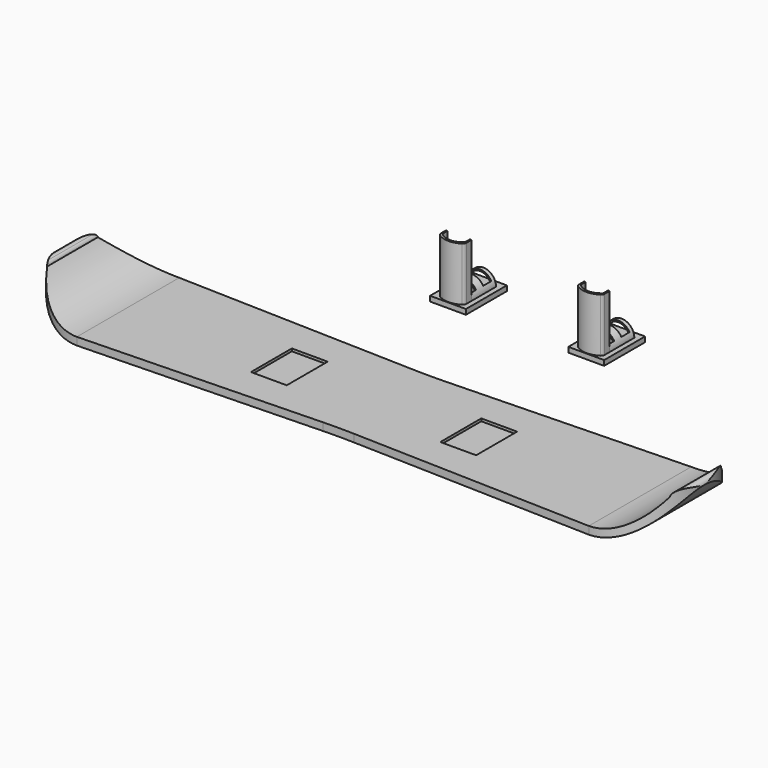
from build123d import *

# Parameters (mm, degrees)
F1_DEPTH    = 9.8425
F3_DEPTH    = 25.4
F5_DEPTH    = 2.667
F6_T1_DEPTH = 0.381
F0_W        = 1.778
F0_H        = 2.54
F0_W_2      = 1.1176
F0_H_2      = 0.508
F0_H_3      = 0.4445
F0_H_4      = 0.2032
F0_W_3      = 0.0762
F0_H_5      = 0.6812858045
F7_DEPTH    = 2.921
F8_DEPTH    = 2.667
F9_DEPTH    = 2.667
F12_DEPTH   = 1.524


# Not quite as in the source:
# - a fillet or chamfer that OpenCascade refuses, or shapes differently, is made with other operations: its cross-section is extruded or revolved along the edge and cut away or added


with BuildPart() as f1:
    # F0 (on Top) → F1 (new body)
    with BuildSketch(Plane.XY):
        with BuildLine():
            Line((-12.7, -6.35), (-12.7, 0))
            ThreePointArc((-12.7, 0), (-15.875, -3.175), (-12.7, -6.35))
        make_face()
        with BuildLine():
            ThreePointArc((12.7, -6.35), (15.875, -3.175), (12.7, 0))
            Line((12.7, 0), (12.7, -6.35))
        make_face()
        Polygon((-6.35, -0.1905), (-12.7, 0), (-12.7, -6.35), (-6.35, -6.1595), (0, -5.969), (6.35, -6.1595), (12.7, -6.35), (12.7, 0), (6.35, -0.1905), (0, -0.381), align=None)
    extrude(amount=-F1_DEPTH)

    # F2 (on Front) → F3 (cut)
    with BuildSketch(Plane.XZ):
        with BuildLine():
            Line((-12.7, -2.54), (0, -2.54))
            Line((0, -2.54), (12.7, -2.54))
            ThreePointArc((12.7, -2.54), (14.2747487895, -2.1336283165), (15.4562218706, -1.016))
            ThreePointArc((15.4562218706, -1.016), (15.4848358871, -0.9182319253), (15.5561717457, -0.8455094828))
            ThreePointArc((15.5561717457, -0.8455094828), (15.745074667, -0.4338744994), (15.875, 0))
            Line((15.875, 0), (-15.875, 0))
            ThreePointArc((-15.875, 0), (-15.7450242413, -0.4340082159), (-15.556034737, -0.8457603215))
            ThreePointArc((-15.556034737, -0.8457603215), (-15.484834563, -0.9183954726), (-15.4562218706, -1.016))
            ThreePointArc((-15.4562218706, -1.016), (-14.2747487895, -2.1336283165), (-12.7, -2.54))
        make_face()
        with BuildLine():
            ThreePointArc((-15.875, -1.016), (-15.7642823045, -0.8395129732), (-15.556034737, -0.8457603215))
            ThreePointArc((-15.556034737, -0.8457603215), (-15.7450242413, -0.4340082159), (-15.875, 0))
            Line((-15.875, 0), (-15.875, -1.016))
        make_face()
        with BuildLine():
            ThreePointArc((-12.7, -2.921), (-14.5513272266, -2.4082120444), (-15.875, -1.016))
            Line((-15.875, -1.016), (-15.875, -9.8425))
            Line((-15.875, -9.8425), (15.875, -9.8425))
            Line((15.875, -9.8425), (15.875, -1.016))
            ThreePointArc((15.875, -1.016), (14.5513272266, -2.4082120444), (12.7, -2.921))
            Line((12.7, -2.921), (0, -2.921))
            Line((0, -2.921), (-12.7, -2.921))
        make_face()
        with BuildLine():
            ThreePointArc((15.875, 0), (15.745074667, -0.4338744994), (15.5561717457, -0.8455094828))
            ThreePointArc((15.5561717457, -0.8455094828), (15.7644251473, -0.8394221507), (15.875, -1.016))
            Line((15.875, -1.016), (15.875, 0))
        make_face()
    extrude(amount=F3_DEPTH, mode=Mode.SUBTRACT)

    # F4 (on Top) → F5 (cut)
    with BuildSketch(Plane.XY):
        Polygon((-3.81, -4.445), (-3.81, -3.175), (-3.81, -1.905), (-5.588, -1.905), (-5.588, -4.445), align=None)
        Polygon((3.81, -1.905), (3.81, -3.175), (3.81, -4.445), (5.588, -4.445), (5.588, -1.905), align=None)
    extrude(amount=-F5_DEPTH, mode=Mode.SUBTRACT)

    # F6: fillet of radius 25.4 on 2 edges, made by hand

    # F6_s2 → F6_t1 (join)
    with BuildSketch(Plane.XY.offset(-2.921)):
        with BuildLine():
            ThreePointArc((-0.7616573313, -5.9918497199), (0, -5.9804274294), (0.7616573313, -5.9918497199))
            Line((0.7616573313, -5.9918497199), (0, -5.969))
            Line((0, -5.969), (-0.7616573313, -5.9918497199))
        make_face()
        with BuildLine():
            ThreePointArc((-0.7616573313, -0.3581502801), (0, -0.3695725706), (0.7616573313, -0.3581502801))
            Line((0.7616573313, -0.3581502801), (0, -0.381))
            Line((0, -0.381), (-0.7616573313, -0.3581502801))
        make_face()
    extrude(amount=F6_T1_DEPTH)


with BuildPart() as f7:
    # F0 (on Top) → F7 (new body)
    with BuildSketch(Plane.XY):
        with Locations((3.429, 6.35)):
            Rectangle(F0_W, F0_H)
        with BuildLine():
            Line((4.064, 6.1127929022), (4.064, 5.4315070978))
            ThreePointArc((4.064, 5.4315070978), (4.0405795527, 5.3399938579), (3.9760769231, 5.2709822559))
            ThreePointArc((3.9760769231, 5.2709822559), (3.429, 5.1111147458), (2.8819230769, 5.2709822559))
            ThreePointArc((2.8819230769, 5.2709822559), (2.8174204473, 5.3399938579), (2.794, 5.4315070978))
            Line((2.794, 5.4315070978), (2.794, 6.1127929022))
            Line((2.794, 6.1127929022), (2.794, 6.5572929022))
            Line((2.794, 6.5572929022), (2.794, 7.0652929022))
            Line((2.794, 7.0652929022), (2.794, 7.2684929022))
            ThreePointArc((2.794, 7.2684929022), (2.8174204473, 7.3600061421), (2.8819230769, 7.4290177441))
            ThreePointArc((2.8819230769, 7.4290177441), (3.429, 7.5888852542), (3.9760769231, 7.4290177441))
            ThreePointArc((3.9760769231, 7.4290177441), (4.0405795527, 7.3600061421), (4.064, 7.2684929022))
            Line((4.064, 7.2684929022), (4.064, 7.0652929022))
            Line((4.064, 7.0652929022), (4.064, 6.5572929022))
            Line((4.064, 6.5572929022), (4.064, 6.1127929022))
        make_face(mode=Mode.SUBTRACT)
        with BuildLine():
            ThreePointArc((2.8702, 5.4315070978), (3.429, 5.2136194824), (3.9878, 5.4315070978))
            Line((3.9878, 5.4315070978), (3.9878, 6.1127929022))
            Line((3.9878, 6.1127929022), (2.8702, 6.1127929022))
            Line((2.8702, 6.1127929022), (2.8702, 5.4315070978))
        make_face()
        with Locations((3.429, 6.8112929022)):
            Rectangle(F0_W_2, F0_H_2)
        with Locations((3.429, 6.3350429022)):
            Rectangle(F0_W_2, F0_H_3)
        with BuildLine():
            Line((3.9878, 7.2684929022), (4.064, 7.2684929022))
            ThreePointArc((4.064, 7.2684929022), (4.0405795527, 7.3600061421), (3.9760769231, 7.4290177441))
            ThreePointArc((3.9760769231, 7.4290177441), (3.429, 7.5888852542), (2.8819230769, 7.4290177441))
            ThreePointArc((2.8819230769, 7.4290177441), (2.8174204473, 7.3600061421), (2.794, 7.2684929022))
            Line((2.794, 7.2684929022), (2.8702, 7.2684929022))
            Line((2.8702, 7.2684929022), (3.9878, 7.2684929022))
        make_face()
        with Locations((3.429, 7.1668929022)):
            Rectangle(F0_W_2, F0_H_4)
        with BuildLine():
            ThreePointArc((3.9760769231, 5.2709822559), (4.0405795527, 5.3399938579), (4.064, 5.4315070978))
            Line((4.064, 5.4315070978), (3.9878, 5.4315070978))
            ThreePointArc((3.9878, 5.4315070978), (3.429, 5.2136194824), (2.8702, 5.4315070978))
            Line((2.8702, 5.4315070978), (2.794, 5.4315070978))
            ThreePointArc((2.794, 5.4315070978), (2.8174204473, 5.3399938579), (2.8819230769, 5.2709822559))
            ThreePointArc((2.8819230769, 5.2709822559), (3.429, 5.1111147458), (3.9760769231, 5.2709822559))
        make_face()
        with Locations((4.0259, 5.77215)):
            Rectangle(F0_W_3, F0_H_5)
        with Locations((2.8321, 5.77215)):
            Rectangle(F0_W_3, F0_H_5)
        with Locations((2.8321, 6.8112929022)):
            Rectangle(F0_W_3, F0_H_2)
        with Locations((4.0259, 6.8112929022)):
            Rectangle(F0_W_3, F0_H_2)
        with Locations((4.0259, 6.3350429022)):
            Rectangle(F0_W_3, F0_H_3)
        with Locations((2.8321, 6.3350429022)):
            Rectangle(F0_W_3, F0_H_3)
        with Locations((2.8321, 7.1668929022)):
            Rectangle(F0_W_3, F0_H_4)
        with Locations((4.0259, 7.1668929022)):
            Rectangle(F0_W_3, F0_H_4)
    extrude(amount=-F7_DEPTH)

    # F0 (on Top) → F9 (cut)
    with BuildSketch(Plane.XY):
        with Locations((3.429, 6.35)):
            Rectangle(F0_W, F0_H)
        with BuildLine():
            Line((4.064, 6.1127929022), (4.064, 5.4315070978))
            ThreePointArc((4.064, 5.4315070978), (4.0405795527, 5.3399938579), (3.9760769231, 5.2709822559))
            ThreePointArc((3.9760769231, 5.2709822559), (3.429, 5.1111147458), (2.8819230769, 5.2709822559))
            ThreePointArc((2.8819230769, 5.2709822559), (2.8174204473, 5.3399938579), (2.794, 5.4315070978))
            Line((2.794, 5.4315070978), (2.794, 6.1127929022))
            Line((2.794, 6.1127929022), (2.794, 6.5572929022))
            Line((2.794, 6.5572929022), (2.794, 7.0652929022))
            Line((2.794, 7.0652929022), (2.794, 7.2684929022))
            ThreePointArc((2.794, 7.2684929022), (2.8174204473, 7.3600061421), (2.8819230769, 7.4290177441))
            ThreePointArc((2.8819230769, 7.4290177441), (3.429, 7.5888852542), (3.9760769231, 7.4290177441))
            ThreePointArc((3.9760769231, 7.4290177441), (4.0405795527, 7.3600061421), (4.064, 7.2684929022))
            Line((4.064, 7.2684929022), (4.064, 7.0652929022))
            Line((4.064, 7.0652929022), (4.064, 6.5572929022))
            Line((4.064, 6.5572929022), (4.064, 6.1127929022))
        make_face(mode=Mode.SUBTRACT)
        with BuildLine():
            ThreePointArc((2.8702, 5.4315070978), (3.429, 5.2136194824), (3.9878, 5.4315070978))
            Line((3.9878, 5.4315070978), (3.9878, 6.1127929022))
            Line((3.9878, 6.1127929022), (2.8702, 6.1127929022))
            Line((2.8702, 6.1127929022), (2.8702, 5.4315070978))
        make_face()
        with Locations((3.429, 6.8112929022)):
            Rectangle(F0_W_2, F0_H_2)
        with BuildLine():
            Line((3.9878, 7.2684929022), (4.064, 7.2684929022))
            ThreePointArc((4.064, 7.2684929022), (4.0405795527, 7.3600061421), (3.9760769231, 7.4290177441))
            ThreePointArc((3.9760769231, 7.4290177441), (3.429, 7.5888852542), (2.8819230769, 7.4290177441))
            ThreePointArc((2.8819230769, 7.4290177441), (2.8174204473, 7.3600061421), (2.794, 7.2684929022))
            Line((2.794, 7.2684929022), (2.8702, 7.2684929022))
            Line((2.8702, 7.2684929022), (3.9878, 7.2684929022))
        make_face()
    extrude(amount=-F9_DEPTH, mode=Mode.SUBTRACT)


with BuildPart() as f7b:
    # F0 (on Top) → F7, piece 2 (new body)
    with BuildSketch(Plane.XY):
        with Locations((-3.429, 6.35)):
            Rectangle(F0_W, F0_H)
        with BuildLine():
            ThreePointArc((-2.8819230769, 5.2709822559), (-3.429, 5.1111147458), (-3.9760769231, 5.2709822559))
            ThreePointArc((-3.9760769231, 5.2709822559), (-4.0405795527, 5.3399938579), (-4.064, 5.4315070978))
            Line((-4.064, 5.4315070978), (-4.064, 6.1127929022))
            Line((-4.064, 6.1127929022), (-4.064, 6.5572929022))
            Line((-4.064, 6.5572929022), (-4.064, 7.0652929022))
            Line((-4.064, 7.0652929022), (-4.064, 7.2684929022))
            ThreePointArc((-4.064, 7.2684929022), (-4.0405795527, 7.3600061421), (-3.9760769231, 7.4290177441))
            ThreePointArc((-3.9760769231, 7.4290177441), (-3.429, 7.5888852542), (-2.8819230769, 7.4290177441))
            ThreePointArc((-2.8819230769, 7.4290177441), (-2.8174204473, 7.3600061421), (-2.794, 7.2684929022))
            Line((-2.794, 7.2684929022), (-2.794, 7.0652929022))
            Line((-2.794, 7.0652929022), (-2.794, 6.5572929022))
            Line((-2.794, 6.5572929022), (-2.794, 6.1127929022))
            Line((-2.794, 6.1127929022), (-2.794, 5.4315070978))
            ThreePointArc((-2.794, 5.4315070978), (-2.8174204473, 5.3399938579), (-2.8819230769, 5.2709822559))
        make_face(mode=Mode.SUBTRACT)
        with BuildLine():
            Line((-3.9878, 6.1127929022), (-3.9878, 5.4315070978))
            ThreePointArc((-3.9878, 5.4315070978), (-3.429, 5.2136194824), (-2.8702, 5.4315070978))
            Line((-2.8702, 5.4315070978), (-2.8702, 6.1127929022))
            Line((-2.8702, 6.1127929022), (-3.9878, 6.1127929022))
        make_face()
        with Locations((-3.429, 6.8112929022)):
            Rectangle(F0_W_2, F0_H_2)
        with Locations((-3.429, 6.3350429022)):
            Rectangle(F0_W_2, F0_H_3)
        with BuildLine():
            ThreePointArc((-3.9760769231, 7.4290177441), (-4.0405795527, 7.3600061421), (-4.064, 7.2684929022))
            Line((-4.064, 7.2684929022), (-3.9878, 7.2684929022))
            Line((-3.9878, 7.2684929022), (-2.8702, 7.2684929022))
            Line((-2.8702, 7.2684929022), (-2.794, 7.2684929022))
            ThreePointArc((-2.794, 7.2684929022), (-2.8174204473, 7.3600061421), (-2.8819230769, 7.4290177441))
            ThreePointArc((-2.8819230769, 7.4290177441), (-3.429, 7.5888852542), (-3.9760769231, 7.4290177441))
        make_face()
        with Locations((-3.429, 7.1668929022)):
            Rectangle(F0_W_2, F0_H_4)
        with BuildLine():
            ThreePointArc((-4.064, 5.4315070978), (-4.0405795527, 5.3399938579), (-3.9760769231, 5.2709822559))
            ThreePointArc((-3.9760769231, 5.2709822559), (-3.429, 5.1111147458), (-2.8819230769, 5.2709822559))
            ThreePointArc((-2.8819230769, 5.2709822559), (-2.8174204473, 5.3399938579), (-2.794, 5.4315070978))
            Line((-2.794, 5.4315070978), (-2.8702, 5.4315070978))
            ThreePointArc((-2.8702, 5.4315070978), (-3.429, 5.2136194824), (-3.9878, 5.4315070978))
            Line((-3.9878, 5.4315070978), (-4.064, 5.4315070978))
        make_face()
        with Locations((-4.0259, 5.77215)):
            Rectangle(F0_W_3, F0_H_5)
        with Locations((-2.8321, 5.77215)):
            Rectangle(F0_W_3, F0_H_5)
        with Locations((-2.8321, 6.8112929022)):
            Rectangle(F0_W_3, F0_H_2)
        with Locations((-4.0259, 6.8112929022)):
            Rectangle(F0_W_3, F0_H_2)
        with Locations((-4.0259, 6.3350429022)):
            Rectangle(F0_W_3, F0_H_3)
        with Locations((-2.8321, 6.3350429022)):
            Rectangle(F0_W_3, F0_H_3)
        with Locations((-4.0259, 7.1668929022)):
            Rectangle(F0_W_3, F0_H_4)
        with Locations((-2.8321, 7.1668929022)):
            Rectangle(F0_W_3, F0_H_4)
    extrude(amount=-F7_DEPTH)

    # F0 (on Top) → F8 (cut)
    with BuildSketch(Plane.XY):
        with Locations((-3.429, 6.35)):
            Rectangle(F0_W, F0_H)
        with BuildLine():
            ThreePointArc((-2.8819230769, 5.2709822559), (-3.429, 5.1111147458), (-3.9760769231, 5.2709822559))
            ThreePointArc((-3.9760769231, 5.2709822559), (-4.0405795527, 5.3399938579), (-4.064, 5.4315070978))
            Line((-4.064, 5.4315070978), (-4.064, 6.1127929022))
            Line((-4.064, 6.1127929022), (-4.064, 6.5572929022))
            Line((-4.064, 6.5572929022), (-4.064, 7.0652929022))
            Line((-4.064, 7.0652929022), (-4.064, 7.2684929022))
            ThreePointArc((-4.064, 7.2684929022), (-4.0405795527, 7.3600061421), (-3.9760769231, 7.4290177441))
            ThreePointArc((-3.9760769231, 7.4290177441), (-3.429, 7.5888852542), (-2.8819230769, 7.4290177441))
            ThreePointArc((-2.8819230769, 7.4290177441), (-2.8174204473, 7.3600061421), (-2.794, 7.2684929022))
            Line((-2.794, 7.2684929022), (-2.794, 7.0652929022))
            Line((-2.794, 7.0652929022), (-2.794, 6.5572929022))
            Line((-2.794, 6.5572929022), (-2.794, 6.1127929022))
            Line((-2.794, 6.1127929022), (-2.794, 5.4315070978))
            ThreePointArc((-2.794, 5.4315070978), (-2.8174204473, 5.3399938579), (-2.8819230769, 5.2709822559))
        make_face(mode=Mode.SUBTRACT)
        with BuildLine():
            Line((-3.9878, 6.1127929022), (-3.9878, 5.4315070978))
            ThreePointArc((-3.9878, 5.4315070978), (-3.429, 5.2136194824), (-2.8702, 5.4315070978))
            Line((-2.8702, 5.4315070978), (-2.8702, 6.1127929022))
            Line((-2.8702, 6.1127929022), (-3.9878, 6.1127929022))
        make_face()
        with Locations((-3.429, 6.8112929022)):
            Rectangle(F0_W_2, F0_H_2)
        with BuildLine():
            ThreePointArc((-3.9760769231, 7.4290177441), (-4.0405795527, 7.3600061421), (-4.064, 7.2684929022))
            Line((-4.064, 7.2684929022), (-3.9878, 7.2684929022))
            Line((-3.9878, 7.2684929022), (-2.8702, 7.2684929022))
            Line((-2.8702, 7.2684929022), (-2.794, 7.2684929022))
            ThreePointArc((-2.794, 7.2684929022), (-2.8174204473, 7.3600061421), (-2.8819230769, 7.4290177441))
            ThreePointArc((-2.8819230769, 7.4290177441), (-3.429, 7.5888852542), (-3.9760769231, 7.4290177441))
        make_face()
    extrude(amount=-F8_DEPTH, mode=Mode.SUBTRACT)


with BuildPart() as f12_tool:
    # F11 (on face) + F10 (on face) → F12 (new body)
    with BuildSketch(Plane(origin=(0, 7.2684929022, 0), x_dir=(-1, 0, 0), z_dir=(0, 1, 0))):
        with BuildLine():
            ThreePointArc((-2.8702, -2.667), (-3.429, -2.1082), (-3.9878, -2.667))
            Line((-3.9878, -2.667), (-2.8702, -2.667))
        make_face()
        with BuildLine():
            Line((-4.064, 0), (-4.064, -2.667))
            ThreePointArc((-4.064, -2.667), (-3.429, -2.032), (-2.794, -2.667))
            Line((-2.794, -2.667), (-2.794, 0))
            Line((-2.794, 0), (-4.064, 0))
        make_face()
    with BuildSketch(Plane(origin=(0, 7.2684929022, 0), x_dir=(-1, 0, 0), z_dir=(0, 1, 0))):
        with BuildLine():
            Line((2.8702, -2.667), (3.9878, -2.667))
            ThreePointArc((3.9878, -2.667), (3.429, -2.1082), (2.8702, -2.667))
        make_face()
        with BuildLine():
            ThreePointArc((2.794, -2.667), (3.429, -2.032), (4.064, -2.667))
            Line((4.064, -2.667), (4.064, 0))
            Line((4.064, 0), (2.794, 0))
            Line((2.794, 0), (2.794, -2.667))
        make_face()
    extrude(amount=-F12_DEPTH)


with BuildPart() as f7_1:
    add(f7.part)

    # F12: cut by f12_tool
    add(f12_tool.part, mode=Mode.SUBTRACT)


with BuildPart() as f7b_1:
    add(f7b.part)

    # F12: cut by f12_tool
    add(f12_tool.part, mode=Mode.SUBTRACT)


solid = Compound([f1.part, f7_1.part, f7b_1.part])
